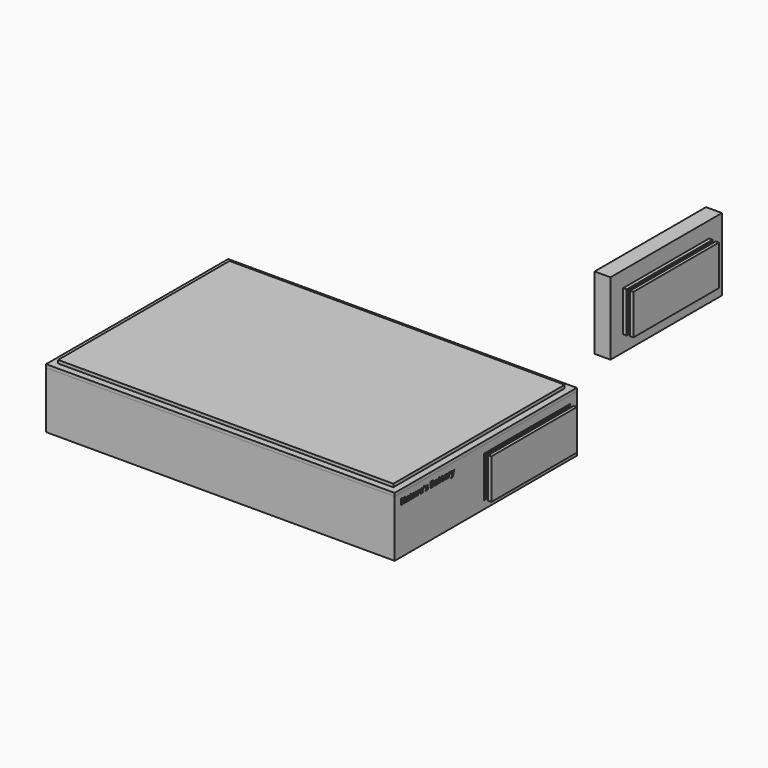
from build123d import *

# Parameters (mm, degrees)
F0_W         = 109.5
F0_H         = 71.5
F1_DEPTH     = 17.8
F2_T         = -2
F3_W         = 109.5
F3_H         = 71.5
F4_DEPTH     = 1
F5_W         = 105.3
F5_H         = 67.3
F6_DEPTH     = 1
F7_W         = 5
F7_H         = 0.3
F8_DEPTH     = 2
F9_TEXT_SIZE = 2.5414525428
F10_DEPTH    = 1
F11_W        = 32.75
F11_H        = 11.8
F12_DEPTH    = 2
F13_W        = 33.95
F13_H        = 13
F14_DEPTH    = 1
F15_W        = 33.75
F15_H        = 12.8
F16_DEPTH    = 1.1
F17_W        = 32.95
F17_H        = 12
F18_DEPTH    = 2
F19_W        = 1
F19_H        = 12
F20_DEPTH    = 0.3
F21_W        = 1
F21_H        = 12
F22_DEPTH    = 0.3
F23_W        = 1
F23_H        = 33.55
F24_DEPTH    = 0.3
F25_W        = 1
F25_H        = 33.55
F26_DEPTH    = 0.3
F27_R        = 2.6
F28_DEPTH    = 1.1
F32_W        = 1
F32_H        = 33.55
F33_DEPTH    = 5
F34_W        = 1
F34_H        = 32.95
F35_DEPTH    = 5.3
F36_W        = 1.1
F36_H        = 33.75
F37_DEPTH    = 4.9
F38_W        = 1
F38_H        = 32.95
F39_DEPTH    = 5.4
F40_W        = 1
F40_H        = 33.55
F41_DEPTH    = 5.1
F42_W        = 1.1
F42_H        = 33.75
F43_DEPTH    = 5
F44_W        = 1
F44_H        = 5.4
F45_DEPTH    = 5.1
F46_W        = 1.1
F46_H        = 5
F47_DEPTH    = 4.9
F48_W        = 1
F48_H        = 5.1
F49_DEPTH    = 4.9
F50_W        = 1
F50_H        = 12.6
F51_DEPTH    = 4.9
F52_W        = 1
F52_H        = 12
F53_DEPTH    = 5
F54_W        = 1.1
F54_H        = 12.8
F55_DEPTH    = 5
F56_W        = 1
F56_H        = 5
F57_DEPTH    = 5
F58_W        = 1
F58_H        = 5.3
F59_DEPTH    = 5
F60_W        = 1.1
F60_H        = 4.9
F61_DEPTH    = 5
F62_W        = 1
F62_H        = 5
F62_H_2      = 17.7167146232
F63_DEPTH    = 5
F64_W        = 1
F64_H        = 22.6877972901
F65_DEPTH    = 5
F66_W        = 1.1
F66_H        = 22.7011510588
F67_DEPTH    = 5
F68_W        = 43.650178954
F68_H        = 22.7033766869
F69_DEPTH    = 5
F74_W        = 33.75
F74_H        = 12.8
F75_DEPTH    = 5
F76_W        = 5
F76_H        = 33.75
F77_DEPTH    = 5
F78_W        = 5
F78_H        = 17.8
F79_DEPTH    = 5
F80_W        = 5
F80_H        = 17.8
F81_DEPTH    = 5
F82_W        = 5
F82_H        = 43.75
F83_DEPTH    = 5


# Not quite as in the source:
# - Text() gives the source's letters only with a copy of the font that has no kerning and outlines rounded to 1/6400 em; it was checked with that copy


with BuildPart() as f1:
    # F0 (on Top) → F1 (new body)
    with BuildSketch(Plane.XY):
        Rectangle(F0_W, F0_H)
    extrude(amount=F1_DEPTH)

    # F2
    f2_openings = [f1.faces().sort_by_distance(p)[0] for p in [
        (0, 0, 17.8),
    ]]
    offset(amount=F2_T, openings=f2_openings)

    # F7 (on face) → F8 (cut)
    with BuildSketch(Plane(origin=(-54.75, 0, 0), x_dir=(0, -1, 0), z_dir=(-1, 0, 0))):
        with Locations((30.75, 2.65)):
            Rectangle(F7_W, F7_H)
        with Locations((30.75, 16.15)):
            Rectangle(F7_W, F7_H)
        with Locations((-30.75, 2.65)):
            Rectangle(F7_W, F7_H)
        with Locations((-30.75, 16.15)):
            Rectangle(F7_W, F7_H)
    extrude(amount=-F8_DEPTH, mode=Mode.SUBTRACT)

    # F9 (on face) → F10 (cut)
    with BuildSketch(Plane.YZ.offset(54.75)):
        with Locations((-33.4913432598, 14.3757257611)):
            Text("Nature's Battery", F9_TEXT_SIZE, font='Open Sans', font_style=FontStyle.BOLD, text_align=(TextAlign.LEFT, TextAlign.BOTTOM))
    extrude(amount=-F10_DEPTH, mode=Mode.SUBTRACT)

    # F11 (on face) → F12 (cut)
    with BuildSketch(Plane.YZ.offset(54.75)):
        with Locations((16.375, 8.9)):
            Rectangle(F11_W, F11_H)
    extrude(amount=-F12_DEPTH, mode=Mode.SUBTRACT)

    # F13 (on face) → F14 (cut)
    with BuildSketch(Plane.YZ.offset(54.75)):
        with Locations((16.375, 8.9)):
            Rectangle(F13_W, F13_H)
    extrude(amount=-F14_DEPTH, mode=Mode.SUBTRACT)

    # F27 (on face) → F28 (cut)
    with BuildSketch(Plane(origin=(-54.75, 0, 0), x_dir=(0, -1, 0), z_dir=(-1, 0, 0))):
        with Locations((-15, 11.245)):
            Circle(F27_R)
        with Locations((15, 11.245)):
            Circle(F27_R)
    extrude(amount=-F28_DEPTH, mode=Mode.SUBTRACT)


with BuildPart() as f4:
    # F3 (on face) → F4 (new body)
    with BuildSketch(Plane.XY.offset(17.8)):
        Rectangle(F3_W, F3_H)
    extrude(amount=F4_DEPTH)

    # F5 (on face) → F6 (join)
    with BuildSketch(Plane.XY.offset(18.8)):
        Rectangle(F5_W, F5_H)
    extrude(amount=F6_DEPTH)


with BuildPart() as f16:
    # F15 (on face) → F16 (new body)
    with BuildSketch(Plane.YZ.offset(53.75)):
        with Locations((16.375, 8.9)):
            Rectangle(F15_W, F15_H)
    extrude(amount=F16_DEPTH)

    # F17 (on face) → F18 (join)
    with BuildSketch(Plane.YZ.offset(54.85)):
        with Locations((16.375, 8.9)):
            Rectangle(F17_W, F17_H)
    extrude(amount=F18_DEPTH)

    # F19 (on face) → F20 (join)
    with BuildSketch(Plane.XZ.offset(0.1)):
        with Locations((56.35, 8.9)):
            Rectangle(F19_W, F19_H)
    extrude(amount=F20_DEPTH)

    # F21 (on face) → F22 (join)
    with BuildSketch(Plane(origin=(0, 32.85, 0), x_dir=(-1, 0, 0), z_dir=(0, 1, 0))):
        with Locations((-56.35, 8.9)):
            Rectangle(F21_W, F21_H)
    extrude(amount=F22_DEPTH)

    # F23 (on face) → F24 (join)
    with BuildSketch(Plane.XY.offset(14.9)):
        with Locations((56.35, 16.375)):
            Rectangle(F23_W, F23_H)
    extrude(amount=F24_DEPTH)

    # F25 (on face) → F26 (join)
    with BuildSketch(Plane(origin=(0, 0, 2.9), x_dir=(1, 0, 0), z_dir=(0, 0, -1))):
        with Locations((56.35, -16.375)):
            Rectangle(F25_W, F25_H)
    extrude(amount=F26_DEPTH)


with BuildPart() as f29_1:
    # F29: copy of F16
    add(f16.part)


with BuildPart() as f31_1:
    # F31: copy of F16
    add(f16.part.moved(Location((76, 0, 0))))


with BuildPart() as f33:
    # F32 (on face) → F33 (new body)
    with BuildSketch(Plane.XY.offset(15.2)):
        with Locations((132.35, 16.375)):
            Rectangle(F32_W, F32_H)
    extrude(amount=F33_DEPTH)


with BuildPart() as f35:
    # F34 (on face) → F35 (new body)
    with BuildSketch(Plane.XY.offset(14.9)):
        with Locations((131.35, 16.375)):
            Rectangle(F34_W, F34_H)
    extrude(amount=F35_DEPTH)


with BuildPart() as f37:
    # F36 (on face) → F37 (new body)
    with BuildSketch(Plane.XY.offset(15.3)):
        with Locations((130.3, 16.375)):
            Rectangle(F36_W, F36_H)
    extrude(amount=F37_DEPTH)


with BuildPart() as f39:
    # F38 (on face) → F39 (new body)
    with BuildSketch(Plane(origin=(0, 0, 2.9), x_dir=(1, 0, 0), z_dir=(0, 0, -1))):
        with Locations((131.35, -16.375)):
            Rectangle(F38_W, F38_H)
    extrude(amount=F39_DEPTH)


with BuildPart() as f41:
    # F40 (on face) → F41 (new body)
    with BuildSketch(Plane(origin=(0, 0, 2.6), x_dir=(1, 0, 0), z_dir=(0, 0, -1))):
        with Locations((132.35, -16.375)):
            Rectangle(F40_W, F40_H)
    extrude(amount=F41_DEPTH)


with BuildPart() as f43:
    # F42 (on face) → F43 (new body)
    with BuildSketch(Plane(origin=(0, 0, 2.5), x_dir=(1, 0, 0), z_dir=(0, 0, -1))):
        with Locations((130.3, -16.375)):
            Rectangle(F42_W, F42_H)
    extrude(amount=F43_DEPTH)


with BuildPart() as f45:
    # F44 (on face) → F45 (new body)
    with BuildSketch(Plane.XZ.offset(0.1)):
        with Locations((131.35, 0.2)):
            Rectangle(F44_W, F44_H)
    extrude(amount=F45_DEPTH)


with BuildPart() as f47:
    # F46 (on face) → F47 (new body)
    with BuildSketch(Plane.XZ.offset(0.5)):
        with Locations((130.3, 0)):
            Rectangle(F46_W, F46_H)
    extrude(amount=F47_DEPTH)


with BuildPart() as f49:
    # F48 (on face) → F49 (new body)
    with BuildSketch(Plane.XZ.offset(0.4)):
        with Locations((132.35, 0.05)):
            Rectangle(F48_W, F48_H)
    extrude(amount=F49_DEPTH)


with BuildPart() as f51:
    # F50 (on face) → F51 (new body)
    with BuildSketch(Plane.XZ.offset(0.4)):
        with Locations((132.35, 8.9)):
            Rectangle(F50_W, F50_H)
    extrude(amount=F51_DEPTH)


with BuildPart() as f53:
    # F52 (on face) → F53 (new body)
    with BuildSketch(Plane.XZ.offset(0.1)):
        with Locations((131.35, 8.9)):
            Rectangle(F52_W, F52_H)
    extrude(amount=F53_DEPTH)


with BuildPart() as f55:
    # F54 (on face) → F55 (new body)
    with BuildSketch(Plane.XZ.offset(0.5)):
        with Locations((130.3, 8.9)):
            Rectangle(F54_W, F54_H)
    extrude(amount=F55_DEPTH)


with BuildPart() as f57:
    # F56 (on face) → F57 (new body)
    with BuildSketch(Plane.XZ.offset(0.4)):
        with Locations((132.35, 17.7)):
            Rectangle(F56_W, F56_H)
    extrude(amount=F57_DEPTH)


with BuildPart() as f59:
    # F58 (on face) → F59 (new body)
    with BuildSketch(Plane.XZ.offset(0.1)):
        with Locations((131.35, 17.55)):
            Rectangle(F58_W, F58_H)
    extrude(amount=F59_DEPTH)


with BuildPart() as f61:
    # F60 (on face) → F61 (new body)
    with BuildSketch(Plane.XZ.offset(0.5)):
        with Locations((130.3, 17.75)):
            Rectangle(F60_W, F60_H)
    extrude(amount=F61_DEPTH)


with BuildPart() as f63:
    # F62 (on face) → F63 (new body)
    with BuildSketch(Plane(origin=(0, 33.15, 0), x_dir=(-1, 0, 0), z_dir=(0, 1, 0))):
        with Locations((-132.35, 17.7)):
            Rectangle(F62_W, F62_H)
        with Locations((-132.35, 6.3416426884)):
            Rectangle(F62_W, F62_H_2)
    extrude(amount=F63_DEPTH)


with BuildPart() as f65:
    # F64 (on face) → F65 (new body)
    with BuildSketch(Plane(origin=(0, 32.85, 0), x_dir=(-1, 0, 0), z_dir=(0, 1, 0))):
        with Locations((-131.35, 8.856101355)):
            Rectangle(F64_W, F64_H)
    extrude(amount=F65_DEPTH)


with BuildPart() as f67:
    # F66 (on face) → F67 (new body)
    with BuildSketch(Plane(origin=(0, 33.25, 0), x_dir=(-1, 0, 0), z_dir=(0, 1, 0))):
        with Locations((-130.3, 8.8494244706)):
            Rectangle(F66_W, F66_H)
    extrude(amount=F67_DEPTH)


with BuildPart() as f69:
    # F68 (on face) → F69 (new body)
    with BuildSketch(Plane(origin=(129.75, 0, 0), x_dir=(0, -1, 0), z_dir=(-1, 0, 0))):
        with Locations((-16.424910523, 8.8483116565)):
            Rectangle(F68_W, F68_H)
    extrude(amount=F69_DEPTH)


with BuildPart() as f73_1:
    # F73: copy of F16
    add(f16.part.moved(Location((44.6, 0, 60))))


with BuildPart() as f75:
    # F74 (on face) → F75 (new body)
    with BuildSketch(Plane(origin=(98.35, 0, 0), x_dir=(0, -1, 0), z_dir=(-1, 0, 0))):
        with Locations((-16.375, 68.9)):
            Rectangle(F74_W, F74_H)
    extrude(amount=F75_DEPTH)

    # F76 (on face) → F77 (join)
    with BuildSketch(Plane.XY.offset(75.3)):
        with Locations((95.85, 16.375)):
            Rectangle(F76_W, F76_H)
    extrude(amount=F77_DEPTH)

    # F78 (on face) → F79 (join)
    with BuildSketch(Plane(origin=(0, 33.25, 0), x_dir=(-1, 0, 0), z_dir=(0, 1, 0))):
        with Locations((-95.85, 71.4)):
            Rectangle(F78_W, F78_H)
    extrude(amount=F79_DEPTH)

    # F80 (on face) → F81 (join)
    with BuildSketch(Plane.XZ.offset(0.5)):
        with Locations((95.85, 71.4)):
            Rectangle(F80_W, F80_H)
    extrude(amount=F81_DEPTH)

    # F82 (on face) → F83 (join)
    with BuildSketch(Plane(origin=(0, 0, 62.5), x_dir=(1, 0, 0), z_dir=(0, 0, -1))):
        with Locations((95.85, -16.375)):
            Rectangle(F82_W, F82_H)
    extrude(amount=F83_DEPTH)


solid = Compound([f1.part, f4.part, f16.part, f73_1.part, f75.part])
